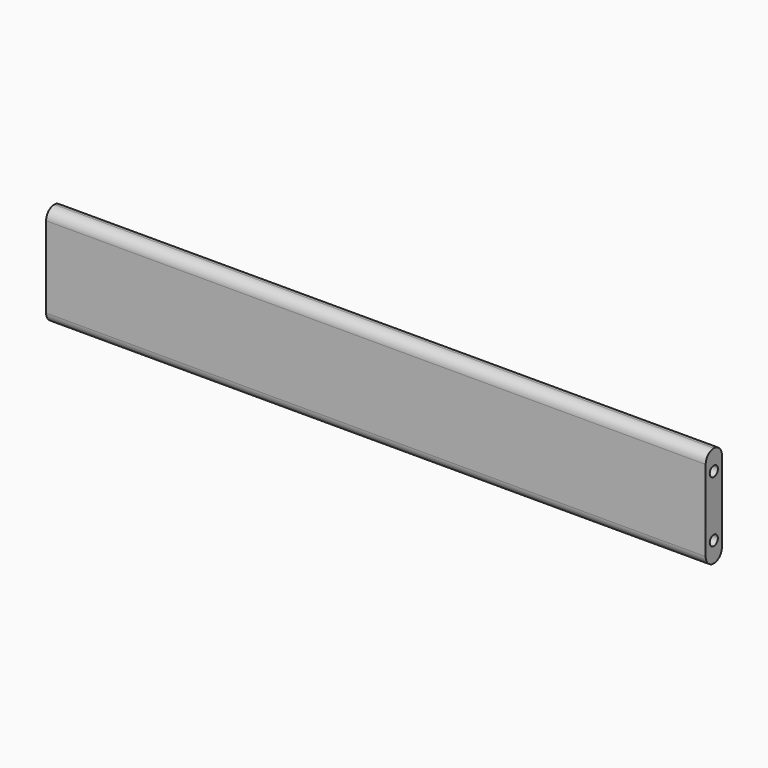
from build123d import *

# Parameters (mm, degrees)
F0_W     = 650
F0_H     = 100
F1_DEPTH = 20
F2_R     = 9.99999
F4_D     = 10
F4_DEPTH = 50
F4_TIP   = 3.0043030951
F6_D     = 10
F6_DEPTH = 50
F6_TIP   = 3.0043030951


# Not quite as in the source:
# - a fillet or chamfer is up to 0.001 mm smaller than in the source, because OpenCascade refuses the exact size


with BuildPart() as f1:
    # F0 (on Front) → F1 (new body)
    with BuildSketch(Plane.XZ):
        with Locations((-325, 50)):
            Rectangle(F0_W, F0_H)
    extrude(amount=F1_DEPTH)

    # F2 (radius 10 in the source; OpenCascade refuses exactly that, so slightly less here)
    f2_edges = [f1.edges().sort_by_distance(p)[0] for p in [
        (-325, 0, 100),
        (-325, -20, 100),
        (-325, 0, 0),
        (-325, -20, 0),
    ]]
    fillet(f2_edges, radius=F2_R)

    # F4
    with Locations(Plane(origin=(-650, 0, 0), x_dir=(0, -1, 0), z_dir=(-1, 0, 0))):
        with Locations((10, 20.0186959194), (10, 80)):
            Hole(F4_D / 2, depth=F4_DEPTH)
            with Locations((0, 0, -(F4_DEPTH + F4_TIP / 2))):  # 118° drill point
                Cone(0, F4_D / 2, F4_TIP, mode=Mode.SUBTRACT)

    # F6
    with Locations(Plane.YZ):
        with Locations((-10, 80), (-10, 20)):
            Hole(F6_D / 2, depth=F6_DEPTH)
            with Locations((0, 0, -(F6_DEPTH + F6_TIP / 2))):  # 118° drill point
                Cone(0, F6_D / 2, F6_TIP, mode=Mode.SUBTRACT)


solid = f1.part
